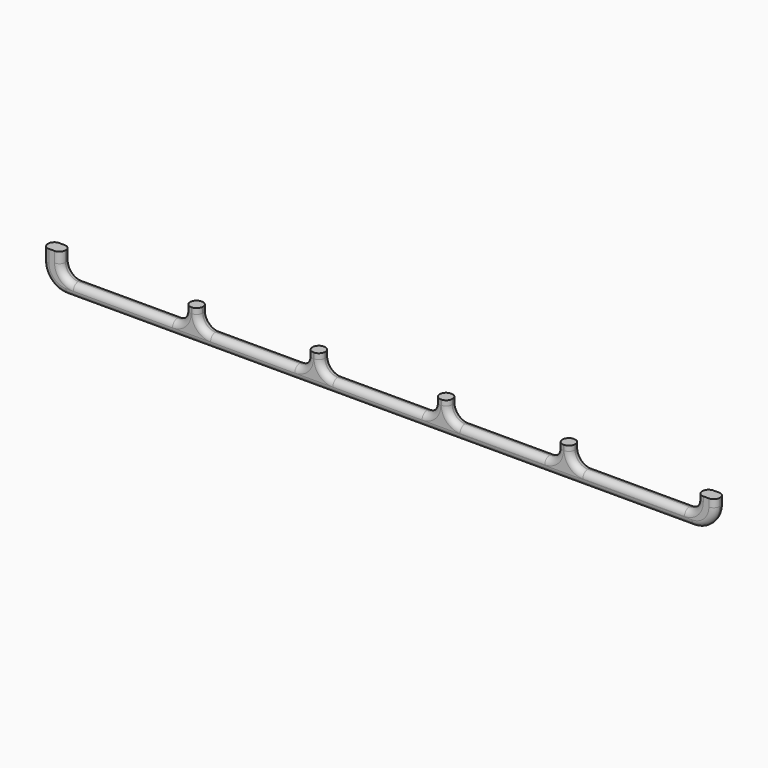
from build123d import *

# Parameters (mm, degrees)
F1_DEPTH = 25
F2_R     = 11.99999


# Not quite as in the source:
# - a fillet or chamfer is up to 0.001 mm smaller than in the source, because OpenCascade refuses the exact size


with BuildPart() as f1:
    # F0 (on Front) → F1 (new body)
    with BuildSketch(Plane.XZ):
        with BuildLine():
            Line((-1280, -60), (-45, -60))
            ThreePointArc((-45, -60), (-13.1801948466, -46.8198051534), (0, -15))
            Line((0, -15), (0, 0))
            Line((0, 0), (-35, 0))
            Line((-35, 0), (-35, -10))
            ThreePointArc((-35, -10), (-42.3223304703, -27.6776695297), (-60, -35))
            Line((-60, -35), (-260.5, -35))
            ThreePointArc((-260.5, -35), (-278.1776695297, -27.6776695297), (-285.5, -10))
            Line((-285.5, -10), (-285.5, 0))
            Line((-285.5, 0), (-310.5, 0))
            Line((-310.5, 0), (-310.5, -10))
            ThreePointArc((-310.5, -10), (-317.8223304703, -27.6776695297), (-335.5, -35))
            Line((-335.5, -35), (-502.5, -35))
            ThreePointArc((-502.5, -35), (-520.1776695297, -27.6776695297), (-527.5, -10))
            Line((-527.5, -10), (-527.5, 0))
            Line((-527.5, 0), (-552.5, 0))
            Line((-552.5, 0), (-552.5, -11))
            ThreePointArc((-552.5, -11), (-559.8223304703, -28.6776695297), (-577.5, -36))
            Line((-577.5, -36), (-753.5, -36))
            ThreePointArc((-753.5, -36), (-771.1776695297, -28.6776695297), (-778.5, -11))
            Line((-778.5, -11), (-778.5, 0))
            Line((-778.5, 0), (-803.5, 0))
            Line((-803.5, 0), (-803.5, -11))
            ThreePointArc((-803.5, -11), (-810.8223304703, -28.6776695297), (-828.5, -36))
            Line((-828.5, -36), (-994.5, -36))
            ThreePointArc((-994.5, -36), (-1012.1776695297, -28.6776695297), (-1019.5, -11))
            Line((-1019.5, -11), (-1019.5, 0))
            Line((-1019.5, 0), (-1044.5, 0))
            Line((-1044.5, 0), (-1044.5, -11))
            ThreePointArc((-1044.5, -11), (-1051.8223304703, -28.6776695297), (-1069.5, -36))
            Line((-1069.5, -36), (-1265, -36))
            ThreePointArc((-1265, -36), (-1282.6776695297, -28.6776695297), (-1290, -11))
            Line((-1290, -11), (-1290, 10))
            Line((-1290, 10), (-1325, 10))
            Line((-1325, 10), (-1325, -15))
            ThreePointArc((-1325, -15), (-1311.8198051534, -46.8198051534), (-1280, -60))
        make_face()
    extrude(amount=F1_DEPTH)

    # F2 (radius 12 in the source; OpenCascade refuses exactly that, so slightly less here)
    f2_edges = [f1.edges().sort_by_distance(p)[0] for p in [
        (-42.32233, 0, -27.67767),
        (-662.5, 0, -60),
        (-317.82233, 0, -27.67767),
        (-559.82233, 0, -28.67767),
        (-810.82233, 0, -28.67767),
        (-1051.82233, 0, -28.67767),
        (-1311.819805, -25, -46.819805),
        (-1282.67767, -25, -28.67767),
        (-911.5, -25, -36),
        (-665.5, -25, -36),
        (-419, -25, -35),
        (-160.25, -25, -35),
    ]]
    fillet(f2_edges, radius=F2_R)


solid = f1.part
